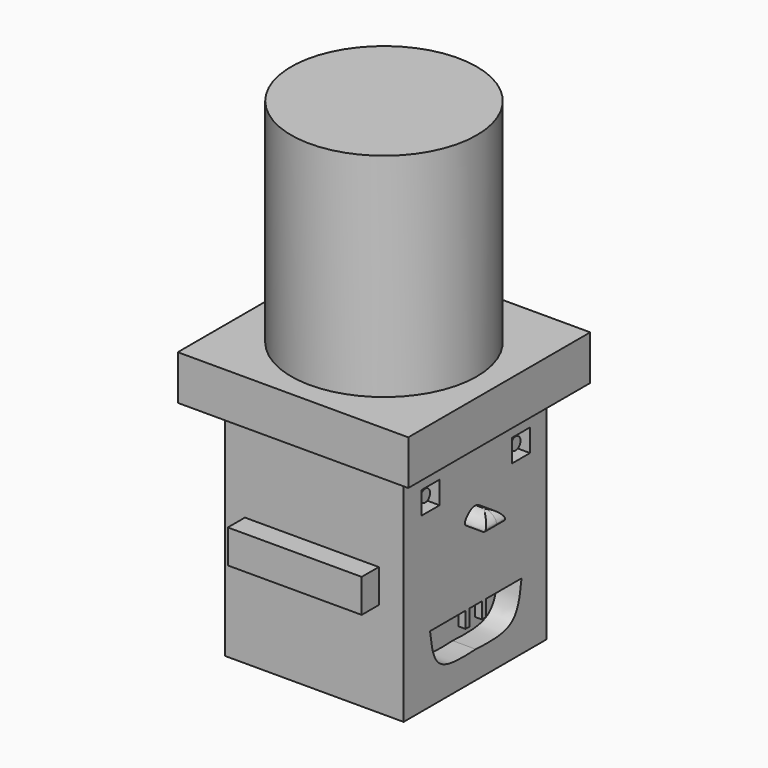
from build123d import *

# Parameters (mm, degrees)
F1_DEPTH      = 63.5
F2_W          = 101.6
F2_H          = 101.6
F3_DEPTH      = 63.5
F4_W          = 12.8822922707
F4_H          = 12.8822997212
F5_DEPTH      = 14.478
F6_R          = 3.4901175811
F7_DEPTH      = 11.43
F9_DEPTH      = 13.208
F10_W         = 3.9928263605
F10_H         = 2.9332810082
F11_DEPTH     = 9.1639515013
F12_W         = 131.2043815851
F12_H         = 129.45997715
F12_W_2       = 101.6
F12_H_2       = 101.6
F13_DEPTH     = 25.4
F14_R         = 52.808946181
F15_DEPTH     = 120.9299713373
F18_DEPTH     = 11.938
F20_DEPTH     = 12.7
F21_TEXT_SIZE = 8.1524573721
F22_DEPTH     = 10.16


# Not quite as in the source:
# - Text() gives the source's letters only with a copy of the font that has no kerning and outlines rounded to 1/6400 em; it was checked with that copy


with BuildPart() as f1:
    # F0 (on Front) → F1 (new body, symmetric)
    with BuildSketch(Plane.XZ):
        Polygon((-38.1, 9.525), (-38.1, -9.525), (38.1, -9.525), (38.1, 9.525), (28.1940001495, 9.525), align=None)
    extrude(amount=F1_DEPTH, both=True)

    # F2 (on Top) → F3 (join, symmetric)
    with BuildSketch(Plane.XY):
        with Locations((1.4337413013, -0.5432718182)):
            Rectangle(F2_W, F2_H)
    extrude(amount=F3_DEPTH, both=True)

    # F4 (on face) → F5 (cut)
    with BuildSketch(Plane.YZ.offset(52.2337413013)):
        with Locations((-32.1806669235, 41.1096736789)):
            Rectangle(F4_W, F4_H)
        with Locations((32.1806669235, 41.1096736789)):
            Rectangle(F4_W, F4_H)
    extrude(amount=-F5_DEPTH, mode=Mode.SUBTRACT)

    # F6 (on face) → F7 (join)
    with BuildSketch(Plane.YZ.offset(37.7557413013)):
        with Locations((32.1806669235, 41.1096736789)):
            Circle(F6_R)
        with Locations((-32.1806669235, 41.1096736789)):
            Circle(F6_R)
    extrude(amount=F7_DEPTH)

    # F8 (on face) → F9 (cut)
    with BuildSketch(Plane.YZ.offset(52.2337413013)):
        with BuildLine():
            add(Edge.make_bspline(
                [(-31.0768830641, -34.6500177945), (-30.5124965587, -36.3513304818), (-29.9288149148, -38.0436443166), (-29.3806409604, -39.7525182013)],
                knots=[1.5909332446, 1.5909332446, 1.5909332446, 1.5909332446, 6.9687199572, 6.9687199572, 6.9687199572, 6.9687199572], degree=3))
            add(Edge.make_bspline(
                [(-29.3806409604, -39.7525182013), (-28.5123273632, -41.6143368382), (-23.3645396187, -48.9364664422), (-10.2443630227, -48.3828122801), (0, -47.9505136609)],
                knots=[0.3166570851, 0.3166570851, 0.3166570851, 0.3166570851, 0.4664391261, 1, 1, 1, 1], degree=3))
            add(Edge.make_bspline(
                [(32.563380897, -25.6479494274), (31.571292663, -33.1370739259), (29.4443522362, -49.1930265225), (10.2443630227, -48.3828122801), (0, -47.9505136609)],
                knots=[0, 0, 0, 0, 0.4664391261, 1, 1, 1, 1], degree=3))
            Line((32.563380897, -25.6479494274), (-32.563380897, -25.6479494274))
            add(Edge.make_bspline(
                [(-32.563380897, -25.6479494274), (-32.1545377196, -28.7342449316), (-31.7456945421, -31.8205404359), (-31.0768830641, -34.6500177945)],
                knots=[0, 0, 0, 0, 0.1922212641, 0.1922212641, 0.1922212641, 0.1922212641], degree=3))
        make_face()
        with BuildLine():
            add(Edge.make_bspline(
                [(-31.0768830641, -34.6500177945), (-30.6439231325, -36.4817003595), (-30.1020179329, -38.205757796), (-29.3806409604, -39.7525182013)],
                knots=[0.1922212641, 0.1922212641, 0.1922212641, 0.1922212641, 0.3166570851, 0.3166570851, 0.3166570851, 0.3166570851], degree=3))
            add(Edge.make_bspline(
                [(-31.0768830641, -34.6500177945), (-30.5124965587, -36.3513304818), (-29.9288149148, -38.0436443166), (-29.3806409604, -39.7525182013)],
                knots=[1.5909332446, 1.5909332446, 1.5909332446, 1.5909332446, 6.9687199572, 6.9687199572, 6.9687199572, 6.9687199572], degree=3))
        make_face()
    extrude(amount=-F9_DEPTH, mode=Mode.SUBTRACT)

    # F10 (on face) → F11 (join)
    with BuildSketch(Plane(origin=(0, 0, -25.6479494274), x_dir=(1, 0, 0), z_dir=(0, 0, -1))):
        with Locations((50.2373281211, 5.8329945896)):
            Rectangle(F10_W, F10_H)
        with Locations((50.2373281211, -5.8329945896)):
            Rectangle(F10_W, F10_H)
    extrude(amount=F11_DEPTH)

    # F12 (on face) → F13 (join)
    with BuildSketch(Plane.XY.offset(63.5)):
        Rectangle(F12_W, F12_H)
        with Locations((1.4337413013, -0.5432718182)):
            Rectangle(F12_W_2, F12_H_2, mode=Mode.SUBTRACT)
        with Locations((1.4337413013, -0.5432718182)):
            Rectangle(F12_W_2, F12_H_2)
    extrude(amount=F13_DEPTH)

    # F14 (on face) → F15 (join)
    with BuildSketch(Plane.XY.offset(88.9)):
        Circle(F14_R)
    extrude(amount=F15_DEPTH)

    # F17 (on face) → F18 (join)
    with BuildSketch(Plane.YZ.offset(52.2337413013)):
        with BuildLine():
            add(Edge.make_bspline(
                [(0, 24.186776951), (-3.601167525, 24.6425071027), (-9.0460677388, 18.663800779), (-6.4339866157, 15.7398011201), (11.6059023274, 13.3825193914), (3.6524269571, 23.7245598839), (0, 24.186776951)],
                knots=[0, 0, 0, 0, 0.270043988, 0.4200888308, 0.7261121748, 1, 1, 1, 1], degree=3))
        make_face()
    extrude(amount=F18_DEPTH)

    # F19 (on Front) → F20 (cut, symmetric)
    with BuildSketch(Plane.XZ):
        with BuildLine():
            Line((52.2337413013, 26.9924197346), (52.2337413013, 24.2239692786))
            add(Edge.make_bspline(
                [(52.2337413013, 24.2239692786), (54.209312334, 24.3871079883), (56.1848833668, 24.550246698), (58.0228277966, 24.2239692786)],
                knots=[0, 0, 0, 0, 0.2209182225, 0.2209182225, 0.2209182225, 0.2209182225], degree=3))
            add(Edge.make_bspline(
                [(58.0228277966, 24.2239692786), (58.9192750317, 24.0648292711), (62.0015606052, 23.0814121223), (66.989615587, 16.6194677434), (57.6958416139, 15.7214787811), (52.2337413013, 15.1937162375)],
                knots=[0.2209182225, 0.2209182225, 0.2209182225, 0.2209182225, 0.3286698642, 0.6054484911, 1, 1, 1, 1], degree=3))
            Line((52.2337413013, 15.1937162375), (52.2337413013, 13.7682445347))
            Line((52.2337413013, 13.7682445347), (68.3657377958, 14.2411142588))
            Line((68.3657377958, 14.2411142588), (68.3657377958, 26.9924197346))
            Line((68.3657377958, 26.9924197346), (52.2337413013, 26.9924197346))
        make_face()
    extrude(amount=F20_DEPTH, both=True, mode=Mode.SUBTRACT)

    # F21 (on face) → F22 (cut)
    with BuildSketch(Plane(origin=(0, 0, -9.525), x_dir=(1, 0, 0), z_dir=(0, 0, -1))):
        with Locations((-30.694811244, -60.96)):
            Text('AIDAN IS DUMB', F21_TEXT_SIZE, font='Open Sans', font_style=FontStyle.BOLD, text_align=(TextAlign.LEFT, TextAlign.BOTTOM))
    extrude(amount=-F22_DEPTH, mode=Mode.SUBTRACT)


solid = f1.part
